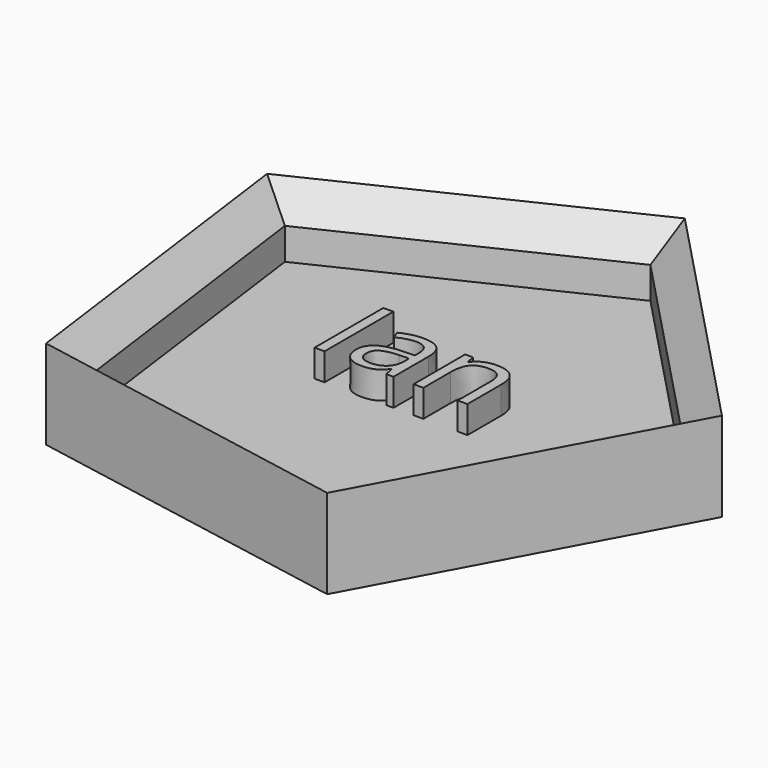
from build123d import *

# Parameters (mm, degrees)
F1_DEPTH     = 15.748
F2_T         = -5.08
F3_SIZE      = 5.07999
F4_TEXT_SIZE = 21.2421220365
F5_DEPTH     = 4.826


# Not quite as in the source:
# - a fillet or chamfer is up to 0.001 mm smaller than in the source, because OpenCascade refuses the exact size
# - Text() gives the source's letters only with a copy of the font that has no kerning and outlines rounded to 1/6400 em; it was checked with that copy


with BuildPart() as f1:
    # F0 (on Top) → F1 (new body)
    with BuildSketch(Plane.XY):
        Polygon((21.7408607147, -45.3218734076), (49.8219584682, 6.6715581527), (9.0508030048, 49.4451231039), (-44.2282545858, 23.8872085034), (-36.3853676018, -34.6820163524), align=None)
    extrude(amount=F1_DEPTH)

    # F2
    f2_openings = [f1.faces().sort_by_distance(p)[0] for p in [
        (0, 0, 15.748),
    ]]
    offset(amount=F2_T, openings=f2_openings)

    # F3 (size 5.08 in the source; OpenCascade refuses exactly that, so slightly less here)
    f3_edges = [f1.edges().sort_by_distance(p)[0] for p in [
        (25.759238, 24.553341, 15.748),
        (-35.271753, -4.723169, 15.748),
        (-15.391572, 32.085891, 15.748),
        (-6.40757, -35.00497, 15.748),
        (31.311657, -16.911092, 15.748),
    ]]
    chamfer(f3_edges, length=F3_SIZE)

    # F4 (on face) → F5 (join)
    with BuildSketch(Plane.XY.offset(5.08)):
        with Locations((-15.7945416868, -3.7824187893)):
            Text('Ian', F4_TEXT_SIZE, font='Open Sans', text_align=(TextAlign.LEFT, TextAlign.BOTTOM))
    extrude(amount=F5_DEPTH)


solid = f1.part
